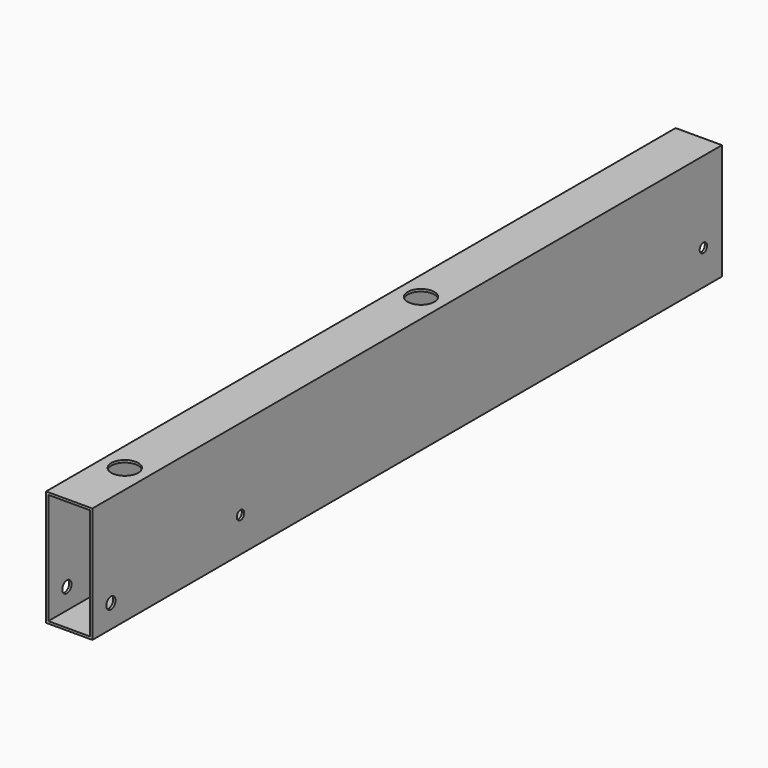
from build123d import *

# Parameters (mm, degrees)
F0_W      = 100
F0_H      = 250
F0_W_2    = 90
F0_H_2    = 240
F1_DEPTH  = 1700
F2_R      = 10
F3_DEPTH  = 100.001
F4_R      = 10
F5_DEPTH  = 100.001
F6_R      = 29
F7_R      = 29
F8_DEPTH  = 5
F9_R      = 12.5
F10_DEPTH = 100.001


# Not quite as in the source:
# - a feature names something its author has since deleted; it is built from what else it names


with BuildPart() as f1:
    # F0 (on Front) → F1 (new body)
    with BuildSketch(Plane.XZ):
        Rectangle(F0_W, F0_H)
        Rectangle(F0_W_2, F0_H_2, mode=Mode.SUBTRACT)
    extrude(amount=F1_DEPTH)

    # F2 (on face) → F3 (cut, through all)
    with BuildSketch(Plane.YZ.offset(50)):
        with Locations((-1300, -50)):
            Circle(F2_R)
    extrude(amount=-F3_DEPTH, mode=Mode.SUBTRACT)

    # F4 (on face) → F5 (cut, through all)
    with BuildSketch(Plane.YZ.offset(50)):
        with Locations((-50, -50)):
            Circle(F4_R)
    extrude(amount=-F5_DEPTH, mode=Mode.SUBTRACT)

    # F6 (on face) + F7 (on face) → F8 (cut, through all)
    with BuildSketch(Plane.XY.offset(125)):
        with Locations((0, -1550)):
            Circle(F6_R)
    with BuildSketch(Plane.XY.offset(125)):
        with Locations((0, -750)):
            Circle(F7_R)
    extrude(amount=-F8_DEPTH, mode=Mode.SUBTRACT)

    # F9 (on face) → F10 (cut, through all)
    with BuildSketch(Plane.YZ.offset(50)):
        with Locations((-1650, -75)):
            Circle(F9_R)
    extrude(amount=-F10_DEPTH, mode=Mode.SUBTRACT)


solid = f1.part
